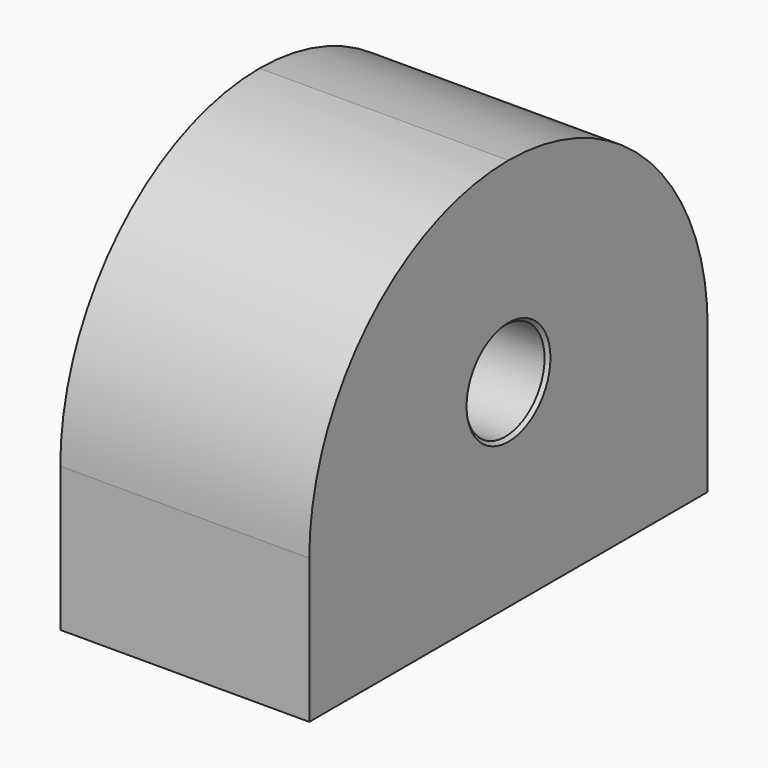
from build123d import *

# Parameters (mm, degrees)
F1_DEPTH = 38
F2_R     = 7.5
F3_DEPTH = 38.001
F4_SIZE  = 0.5
F5_R     = 5
F6_DEPTH = 13
F7_SIZE  = 0.5


# Not quite as in the source:
# - a feature names something its author has since deleted; it is built from what else it names


with BuildPart() as f1:
    # F0 (on Right) → F1 (new body)
    with BuildSketch(Plane.YZ):
        with BuildLine():
            Line((-38, 0), (0, 0))
            Line((0, 0), (38, 0))
            Line((38, 0), (38, 22))
            ThreePointArc((38, 22), (26.8700576851, 48.8700576851), (0, 60))
            ThreePointArc((0, 60), (-26.8700576851, 48.8700576851), (-38, 22))
            Line((-38, 22), (-38, 0))
        make_face()
    extrude(amount=-F1_DEPTH)

    # F2 (on face) → F3 (cut, through all)
    with BuildSketch(Plane.YZ):
        with Locations((0, 30.2)):
            Circle(F2_R)
    extrude(amount=-F3_DEPTH, mode=Mode.SUBTRACT)

    # F4
    f4_edges = [f1.edges().sort_by_distance(p)[0] for p in [
        (0, -7.5, 30.2),
        (-19, 7.5, 30.2),
        (-38, -7.5, 30.2),
    ]]
    chamfer(f4_edges, length=F4_SIZE)

    # F5 (on face) → F6 (cut)
    with BuildSketch(Plane(origin=(0, 0, 0), x_dir=(1, 0, 0), z_dir=(0, 0, -1))):
        with Locations((-19, 29.5)):
            Circle(F5_R)
        with Locations((-19, -29.5)):
            Circle(F5_R)
    extrude(amount=-F6_DEPTH, mode=Mode.SUBTRACT)

    # F7
    f7_edges = [f1.edges().sort_by_distance(p)[0] for p in [
        (-14, -29.5, 6.5),
        (-24, -29.5, 0),
        (-24, -29.5, 13),
        (-14, 29.5, 6.5),
        (-24, 29.5, 0),
        (-24, 29.5, 13),
    ]]
    chamfer(f7_edges, length=F7_SIZE)


solid = f1.part
